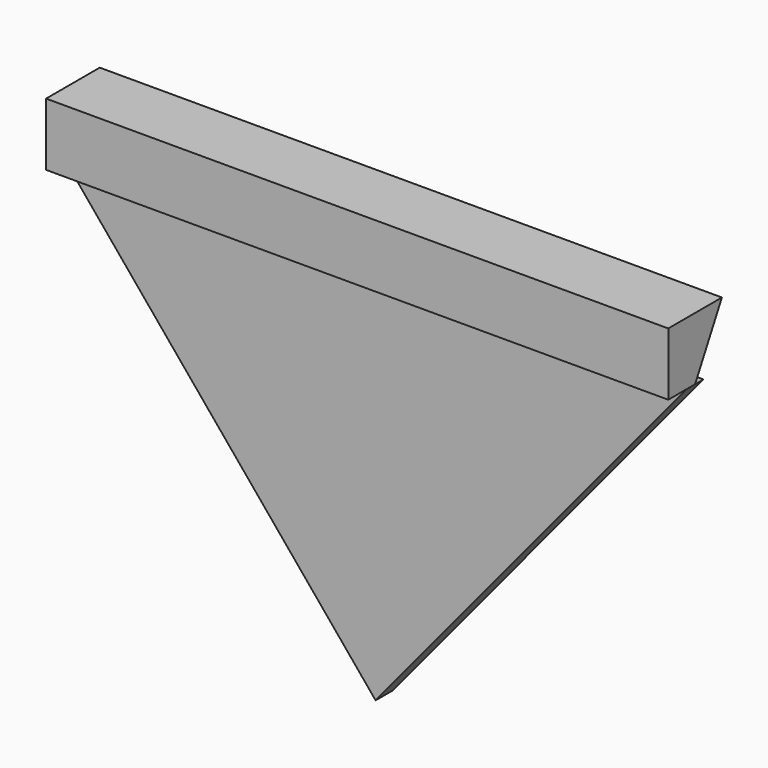
from build123d import *

# Parameters (mm, degrees)
F0_W     = 18.8512783498
F0_H     = 1.9018952735
F1_DEPTH = 1.016
F2_DEPTH = 0.3175
F4_DEPTH = 50.8


with BuildPart() as f1:
    # F0 (on Front) → F1 (new body, symmetric)
    with BuildSketch(Plane.XZ):
        with Locations((9.4256391749, -0.9509476367)):
            Rectangle(F0_W, F0_H)
    extrude(amount=F1_DEPTH, both=True)

    # F0 (on Front) → F2 (join, symmetric)
    with BuildSketch(Plane.XZ):
        with Locations((9.4256391749, -0.9509476367)):
            Rectangle(F0_W, F0_H)
        Polygon((18.8512783498, -1.9018952735), (0, -1.9018952735), (9.4256391749, -13.2702235132), align=None)
    extrude(amount=F2_DEPTH, both=True)

    # F3 (on face) → F4 (cut, symmetric)
    with BuildSketch(Plane.YZ.offset(18.8512783498)):
        Polygon((1.016, -1.9018952735), (1.016, 0), (0, -1.9018952735), (0.3175, -1.9018952735), align=None)
    extrude(amount=F4_DEPTH, both=True, mode=Mode.SUBTRACT)


solid = f1.part
